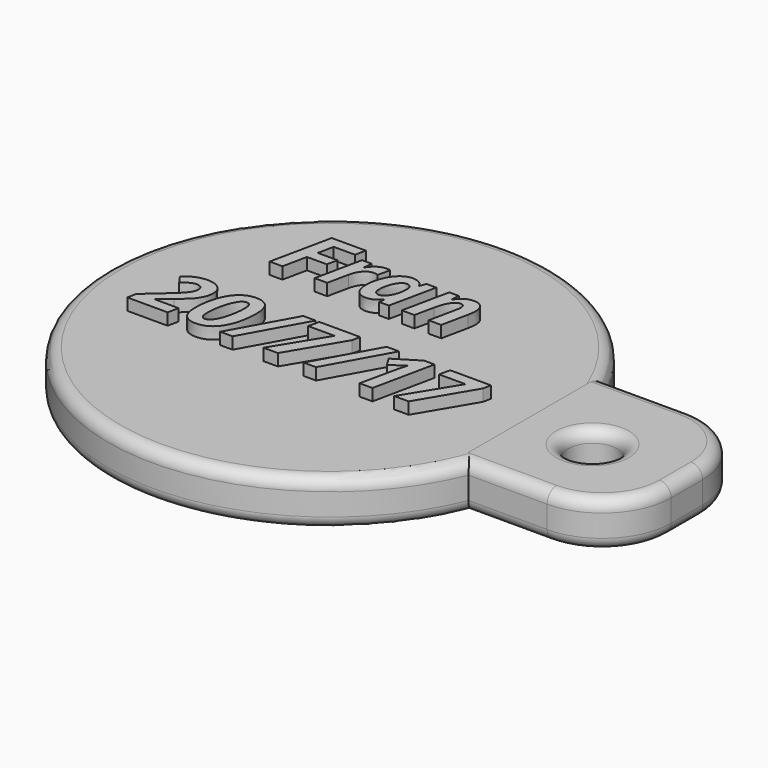
from build123d import *

# Parameters (mm, degrees)
F0_W         = 11.265
F0_H         = 2.33
F2_TEXT_SIZE = 4.3645557111
F3_DEPTH     = 0.6
F4_W         = 8
F4_H         = 9
F5_DEPTH     = 2.33
F6_R         = 1.2430676512
F7_DEPTH     = 2.331
F8_R         = 3.5
F9_R         = 0.6
F9_2_R       = 0.6


# Not quite as in the source:
# - Text() gives the source's letters only with a copy of the font that has no kerning and outlines rounded to 1/6400 em; it was checked with that copy


with BuildPart() as f1:
    # F0 (on Front) → F1 (revolve)
    with BuildSketch(Plane.XZ):
        with Locations((5.6325, 1.165)):
            Rectangle(F0_W, F0_H)
    revolve(axis=Axis((0, 0, 1.165), (0, 0, -1)))

    # F2 (on face) → F3 (join)
    with BuildSketch(Plane.XY.offset(2.33)):
        with Locations((-5.8672586032, 3.3597179023)):
            Text('Fran', F2_TEXT_SIZE, font='Open Sans', font_style=FontStyle.BOLDITALIC, text_align=(TextAlign.LEFT, TextAlign.BOTTOM))
        with Locations((-8.1354636494, -2.5760778648)):
            Text('20/7/17', F2_TEXT_SIZE, font='Open Sans', font_style=FontStyle.BOLDITALIC, text_align=(TextAlign.LEFT, TextAlign.BOTTOM))
    extrude(amount=F3_DEPTH)

    # F9
    f9_edges = [f1.edges().sort_by_distance(p)[0] for p in [
        (-11.265, 0, 2.33),
        (-11.265, 0, 0),
    ]]
    fillet(f9_edges, radius=F9_R)


with BuildPart() as f5:
    # F4 (on Top) → F5 (new body)
    with BuildSketch(Plane.XY):
        with Locations((13.9281972013, 0.2581963433)):
            Rectangle(F4_W, F4_H)
    extrude(amount=F5_DEPTH)

    # F6 (on face) → F7 (cut, through all)
    with BuildSketch(Plane.XY.offset(2.33)):
        with Locations((13.3375991136, 0)):
            Circle(F6_R)
    extrude(amount=-F7_DEPTH, mode=Mode.SUBTRACT)

    # F8
    f8_edges = [f5.edges().sort_by_distance(p)[0] for p in [
        (17.928197, -4.241804, 1.165),
        (17.928197, 4.758196, 1.165),
    ]]
    fillet(f8_edges, radius=F8_R)

    # F9#2
    f9_2_edges = [f5.edges().sort_by_distance(p)[0] for p in [
        (12.178197, -4.241804, 2.33),
        (16.903071, -3.216677, 2.33),
        (17.928197, 0.258196, 2.33),
        (16.903071, 3.73307, 2.33),
        (12.178197, -4.241804, 0),
        (16.903071, -3.216677, 0),
        (17.928197, 0.258196, 0),
        (16.903071, 3.73307, 0),
        (12.178197, 4.758196, 2.33),
        (12.094531, 0, 2.33),
        (12.178197, 4.758196, 0),
        (12.094531, 0, 0),
    ]]
    fillet(f9_2_edges, radius=F9_2_R)


solid = Compound([f1.part, f5.part])
